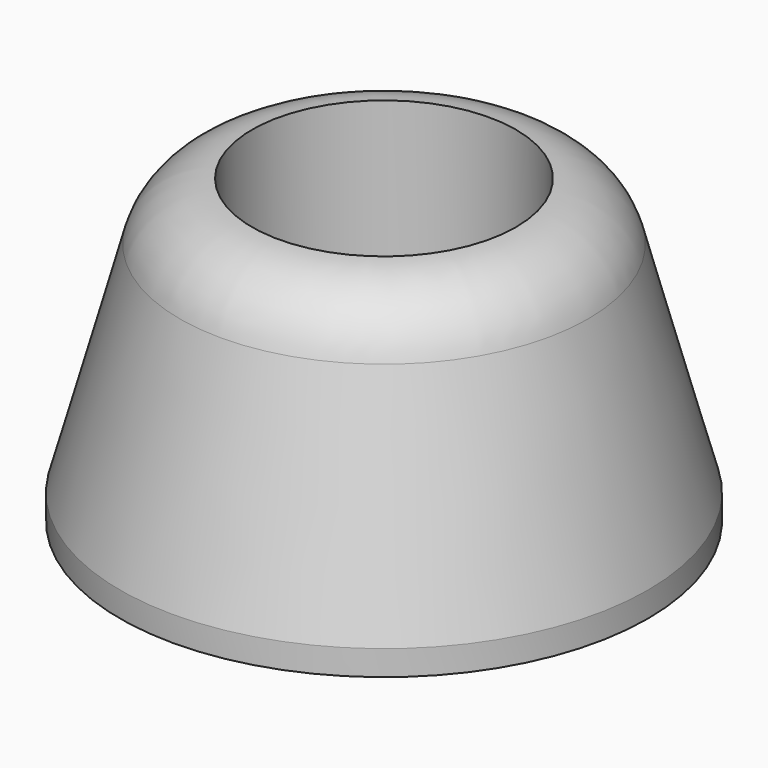
from build123d import *

# Parameters (mm, degrees)
F0_R      = 10.5
F1_DEPTH  = 1
F1_FACE_R = 10.5
F3_R      = 7.5
F5_R      = 2.5
F6_DEPTH  = 12
F7_R      = 5.25
F8_DEPTH  = 10


# Not quite as in the source:
# - a fillet or chamfer that OpenCascade refuses, or shapes differently, is made with other operations: its cross-section is extruded or revolved along the edge and cut away or added


with BuildPart() as f1:
    # F0 (on Top) → F1 (new body)
    with BuildSketch(Plane.XY):
        Circle(F0_R)
    extrude(amount=F1_DEPTH)

    # F1_face (on face) → F4 section 0
    with BuildSketch(Plane.XY.offset(1)):
        Circle(F1_FACE_R)
    # F3 (on offset) → F4 section 1
    with BuildSketch(Plane.XY.offset(12)):
        Circle(F3_R)
    loft()

    # F5 (on Top) → F6 (cut, through all)
    with BuildSketch(Plane.XY):
        Circle(F5_R)
    extrude(amount=F6_DEPTH, mode=Mode.SUBTRACT)

    # F7 (on offset) → F8 (cut)
    with BuildSketch(Plane.XY.offset(12)):
        Circle(F7_R)
    extrude(amount=-F8_DEPTH, mode=Mode.SUBTRACT)

    # F9: fillet of radius 3.0968632265 on 1 edges, made by hand

    # F9_s1 → F9_t2 (revolve, cut)
    with BuildSketch(Plane.XZ):
        with BuildLine():
            ThreePointArc((8.1217780062, 9.7201473108), (7.0595697228, 11.3307742745), (5.25, 12))
            Line((5.25, 12), (7.5, 12))
            Line((7.5, 12), (8.1217780062, 9.7201473108))
        make_face()
    revolve(axis=Axis((0, 0, 12), (0, 0, 1)), mode=Mode.SUBTRACT)


solid = f1.part
